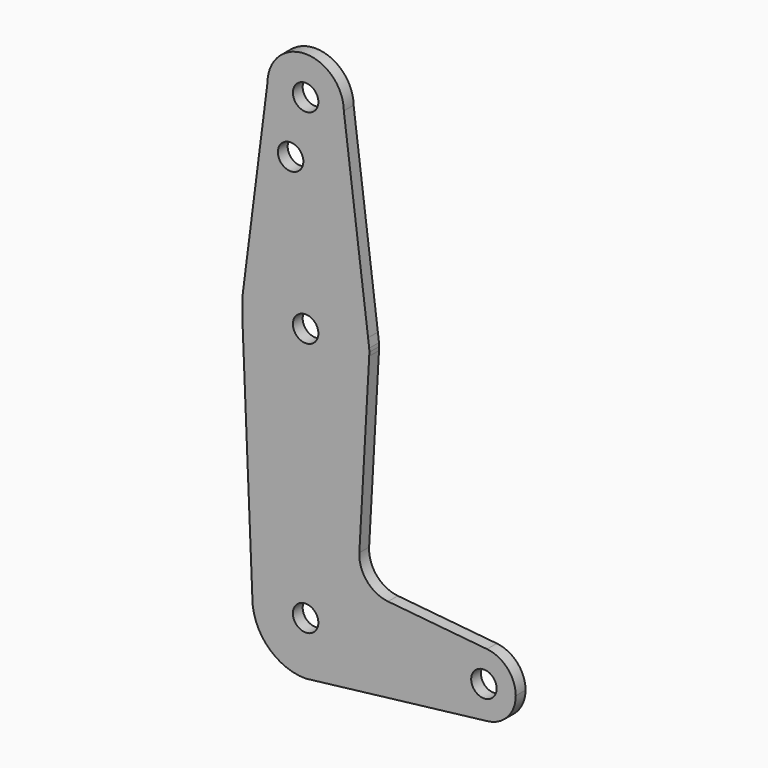
from build123d import *

# Parameters (mm, degrees)
F0_R     = 3.175
F1_DEPTH = 3.048


with BuildPart() as f1:
    # F0 (on Front) → F1 (new body)
    with BuildSketch(Plane.XZ):
        with BuildLine():
            ThreePointArc((3.1097588161, -12.904249902), (10.427563759, -8.2131710978), (13.2736681226, 0))
            ThreePointArc((13.2736681226, 0), (0, 13.2736681226), (-13.2736681226, 0))
            ThreePointArc((-13.2736681226, 0), (-9.3859007407, -9.3859007407), (0, -13.2736681226))
            Line((0, -13.2736681226), (3.1097588161, -12.904249902))
        make_face()
        Circle(F0_R, mode=Mode.SUBTRACT)
        with BuildLine():
            ThreePointArc((-13.2736681226, 0), (0, 13.2736681226), (13.2736681226, 0))
            ThreePointArc((13.2736681226, 0), (10.427563759, -8.2131710978), (3.1097588161, -12.904249902))
            Line((3.1097588161, -12.904249902), (45.3863375042, -7.8820795688))
            ThreePointArc((45.3863375042, -7.8820795688), (36.5129073275, -0.0804124208), (45.2264515588, 7.8994322091))
            Line((45.2264515588, 7.8994322091), (20.5507771811, 10.3248553698))
            ThreePointArc((20.5507771811, 10.3248553698), (15.2912984453, 13.0640911975), (13.39070093, 18.6813199251))
            Line((13.39070093, 18.6813199251), (15.8501799769, 62.6126332776))
            ThreePointArc((15.8501799769, 62.6126332776), (0.5628098086, 47.6349796685), (-15.7474569047, 61.4917106696))
            Line((-15.7474569047, 61.4917106696), (-15.7474569047, 60.0759088993))
            Line((-15.7474569047, 60.0759088993), (-13.2736681226, 0))
        make_face()
        with BuildLine():
            ThreePointArc((45.2264515588, 7.8994322091), (36.5129073275, -0.0804124208), (45.3863375042, -7.8820795688))
            ThreePointArc((45.3863375042, -7.8820795688), (50.3844791342, -5.2712298048), (52.3875, 0))
            ThreePointArc((52.3875, 0), (50.3307733547, 5.3310797219), (45.2264515588, 7.8994322091))
        make_face()
        with Locations((44.45, 0)):
            Circle(F0_R, mode=Mode.SUBTRACT)
        with BuildLine():
            Line((-15.7474569047, 65.5082893304), (-15.7474569047, 61.4917106696))
            ThreePointArc((-15.7474569047, 61.4917106696), (0.5628098086, 47.6349796685), (15.8501799769, 62.6126332776))
            ThreePointArc((15.8501799769, 62.6126332776), (15.8687937811, 63.0561431161), (15.875, 63.5))
            ThreePointArc((15.875, 63.5), (15.8687937811, 63.9438568839), (15.8501799769, 64.3873667224))
            Line((15.8501799769, 64.3873667224), (15.5721686032, 66.5859666221))
            ThreePointArc((15.5721686032, 66.5859666221), (-0.5459199423, 79.3656104962), (-15.7474569047, 65.5082893304))
        make_face()
        with Locations((0, 63.5)):
            Circle(F0_R, mode=Mode.SUBTRACT)
        with BuildLine():
            Line((-9.525, 114.3), (-15.7474569047, 65.5082893304))
            ThreePointArc((-15.7474569047, 65.5082893304), (-0.5459199423, 79.3656104962), (15.5721686032, 66.5859666221))
            Line((15.5721686032, 66.5859666221), (9.5243145818, 114.4142661242))
            ThreePointArc((9.5243145818, 114.4142661242), (9.5248286439, 114.3571340899), (9.525, 114.3))
            ThreePointArc((9.525, 114.3), (0, 104.775), (-9.525, 114.3))
        make_face()
        with Locations((-3.7440145388, 100.0252)):
            Circle(F0_R, mode=Mode.SUBTRACT)
        with BuildLine():
            ThreePointArc((9.5243145818, 114.4142661242), (-0.0571340899, 123.8248286439), (-9.525, 114.3))
            ThreePointArc((-9.525, 114.3), (0, 104.775), (9.525, 114.3))
            ThreePointArc((9.525, 114.3), (9.5248286439, 114.3571340899), (9.5243145818, 114.4142661242))
        make_face()
        with Locations((0, 114.3)):
            Circle(F0_R, mode=Mode.SUBTRACT)
    extrude(amount=F1_DEPTH)


solid = f1.part
